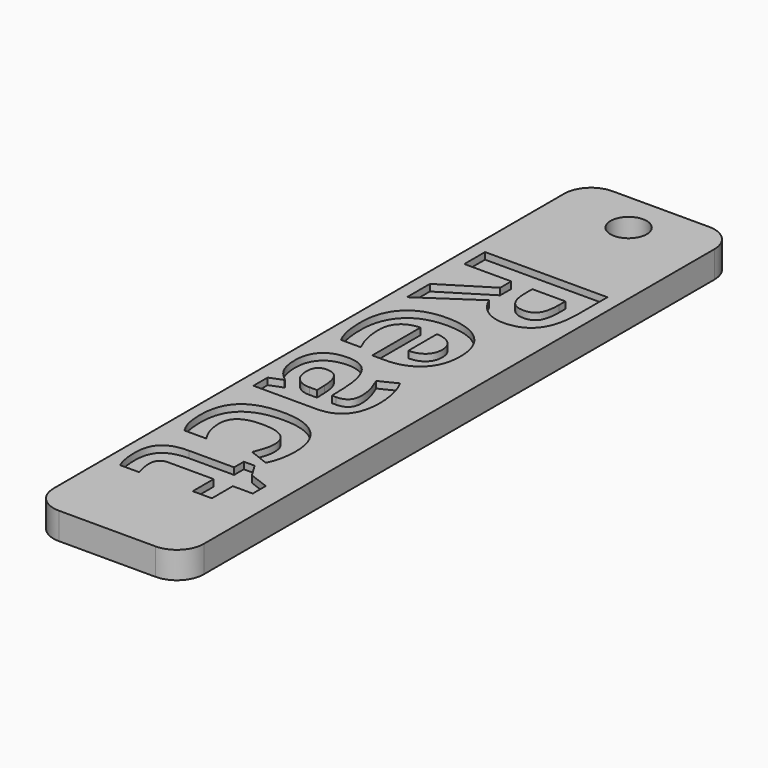
from build123d import *

# Parameters (mm, degrees)
F0_W         = 11.2
F0_H         = 51.6
F0_R         = 1.35
F0_TEXT_SIZE = 12.7777777778
F1_DEPTH     = 2
F2_DEPTH     = 0.5
F3_R         = 2


# Not quite as in the source:
# - Text() gives the source's letters only with a copy of the font that has no kerning and outlines rounded to 1/6400 em; it was checked with that copy


with BuildPart() as f1:
    # F0 (on Top) → F1 (new body)
    with BuildSketch(Plane.XY):
        with Locations((-43.6647401989, 48.8220913022)):
            Rectangle(F0_W, F0_H)
        with BuildLine():
            add(Edge.make_bspline(
                [(-46.6794971433, 31.5330288022), (-46.8731603377, 31.3054246355), (-46.8731603377, 30.9300774133)],
                knots=[0, 0, 0, 1, 1, 1], degree=2))
            add(Edge.make_bspline(
                [(-46.8731603377, 30.9300774133), (-46.8731603377, 30.4309454688), (-46.65553881, 29.7321607466)],
                knots=[0, 0, 0, 1, 1, 1], degree=2))
            Line((-46.65553881, 29.7321607466), (-48.0710770044, 29.7321607466))
            add(Edge.make_bspline(
                [(-48.0710770044, 29.7321607466), (-48.3905214489, 30.4429246355), (-48.3905214489, 31.4791225522)],
                knots=[0, 0, 0, 1, 1, 1], degree=2))
            add(Edge.make_bspline(
                [(-48.3905214489, 31.4791225522), (-48.3905214489, 32.6211364411), (-47.8125266572, 33.1422301911)],
                knots=[0, 0, 0, 1, 1, 1], degree=2))
            add(Edge.make_bspline(
                [(-47.8125266572, 33.1422301911), (-47.2345318655, 33.6633239411), (-46.08053881, 33.6633239411)],
                knots=[0, 0, 0, 1, 1, 1], degree=2))
            Line((-46.08053881, 33.6633239411), (-42.7183860322, 33.6633239411))
            Line((-42.7183860322, 33.6633239411), (-42.7183860322, 34.5737406077))
            Line((-42.7183860322, 34.5737406077), (-41.9137853377, 34.5737406077))
            Line((-41.9137853377, 34.5737406077), (-41.2768929766, 33.5255635244))
            Line((-41.2768929766, 33.5255635244), (-39.8034554766, 32.9765183855))
            Line((-39.8034554766, 32.9765183855), (-39.8034554766, 31.7606329688))
            Line((-39.8034554766, 31.7606329688), (-41.2888721433, 31.7606329688))
            Line((-41.2888721433, 31.7606329688), (-41.2888721433, 29.8080288022))
            Line((-41.2888721433, 29.8080288022), (-42.7183860322, 29.8080288022))
            Line((-42.7183860322, 29.8080288022), (-42.7183860322, 31.7606329688))
            Line((-42.7183860322, 31.7606329688), (-46.08053881, 31.7606329688))
            add(Edge.make_bspline(
                [(-46.08053881, 31.7606329688), (-46.4858339489, 31.7606329688), (-46.6794971433, 31.5330288022)],
                knots=[0, 0, 0, 1, 1, 1], degree=2))
        make_face(mode=Mode.SUBTRACT)
        with BuildLine():
            add(Edge.make_bspline(
                [(-48.2777176294, 36.4185322744), (-48.3905214489, 36.88971283), (-48.3905214489, 37.6064663022)],
                knots=[0, 0, 0, 1, 1, 1], degree=2))
            add(Edge.make_bspline(
                [(-48.3905214489, 37.6064663022), (-48.3905214489, 40.8628031077), (-44.8147401989, 40.8628031077)],
                knots=[0, 0, 0, 1, 1, 1], degree=2))
            add(Edge.make_bspline(
                [(-44.8147401989, 40.8628031077), (-43.0358339489, 40.8628031077), (-42.0974658933, 39.9773430383)],
                knots=[0, 0, 0, 1, 1, 1], degree=2))
            add(Edge.make_bspline(
                [(-42.0974658933, 39.9773430383), (-41.1590978377, 39.0918829688), (-41.1590978377, 37.4387579688)],
                knots=[0, 0, 0, 1, 1, 1], degree=2))
            add(Edge.make_bspline(
                [(-41.1590978377, 37.4387579688), (-41.1590978377, 36.2288621355), (-41.6322749211, 35.2665357466)],
                knots=[0, 0, 0, 1, 1, 1], degree=2))
            Line((-41.6322749211, 35.2665357466), (-43.1057124211, 35.82955658))
            add(Edge.make_bspline(
                [(-43.1057124211, 35.82955658), (-42.9240283933, 36.27877533), (-42.8082297822, 36.665103455)],
                knots=[0, 0, 0, 1, 1, 1], degree=2))
            add(Edge.make_bspline(
                [(-42.8082297822, 36.665103455), (-42.6924311711, 37.05143158), (-42.6924311711, 37.4387579688)],
                knots=[0, 0, 0, 1, 1, 1], degree=2))
            add(Edge.make_bspline(
                [(-42.6924311711, 37.4387579688), (-42.6924311711, 38.9241746355), (-44.8027610322, 38.9241746355)],
                knots=[0, 0, 0, 1, 1, 1], degree=2))
            add(Edge.make_bspline(
                [(-44.8027610322, 38.9241746355), (-46.8492020044, 38.9241746355), (-46.8492020044, 37.4387579688)],
                knots=[0, 0, 0, 1, 1, 1], degree=2))
            add(Edge.make_bspline(
                [(-46.8492020044, 37.4387579688), (-46.8492020044, 36.88971283), (-46.7024572127, 36.4215270661)],
                knots=[0, 0, 0, 1, 1, 1], degree=2))
            add(Edge.make_bspline(
                [(-46.7024572127, 36.4215270661), (-46.5557124211, 35.9533413022), (-46.24225756, 35.4861538022)],
                knots=[0, 0, 0, 1, 1, 1], degree=2))
            Line((-46.24225756, 35.4861538022), (-47.8714242266, 35.4861538022))
            add(Edge.make_bspline(
                [(-47.8714242266, 35.4861538022), (-48.16491381, 35.9473517188), (-48.2777176294, 36.4185322744)],
                knots=[0, 0, 0, 1, 1, 1], degree=2))
        make_face(mode=Mode.SUBTRACT)
        with BuildLine():
            Line((-48.2647401989, 42.4001294966), (-48.2647401989, 43.7278204688))
            Line((-48.2647401989, 43.7278204688), (-47.3163895044, 44.0971781077))
            Line((-47.3163895044, 44.0971781077), (-47.3163895044, 44.1470913022))
            add(Edge.make_bspline(
                [(-47.3163895044, 44.1470913022), (-47.9213374211, 44.6262579688), (-48.155929435, 45.1353725522)],
                knots=[0, 0, 0, 1, 1, 1], degree=2))
            add(Edge.make_bspline(
                [(-48.155929435, 45.1353725522), (-48.3905214489, 45.6444871355), (-48.3905214489, 46.4610669966)],
                knots=[0, 0, 0, 1, 1, 1], degree=2))
            add(Edge.make_bspline(
                [(-48.3905214489, 46.4610669966), (-48.3905214489, 47.4653204688), (-47.8155214489, 48.0423169966)],
                knots=[0, 0, 0, 1, 1, 1], degree=2))
            add(Edge.make_bspline(
                [(-47.8155214489, 48.0423169966), (-47.2405214489, 48.6193135244), (-46.1803651989, 48.6193135244)],
                knots=[0, 0, 0, 1, 1, 1], degree=2))
            add(Edge.make_bspline(
                [(-46.1803651989, 48.6193135244), (-45.0702957544, 48.6193135244), (-44.5432124211, 47.8426642188)],
                knots=[0, 0, 0, 1, 1, 1], degree=2))
            add(Edge.make_bspline(
                [(-44.5432124211, 47.8426642188), (-44.0161290877, 47.0660149133), (-43.96022631, 45.5007371355)],
                knots=[0, 0, 0, 1, 1, 1], degree=2))
            Line((-43.96022631, 45.5007371355), (-43.9222922822, 44.2888447744))
            Line((-43.9222922822, 44.2888447744), (-43.6168235322, 44.2888447744))
            add(Edge.make_bspline(
                [(-43.6168235322, 44.2888447744), (-42.5566672822, 44.2888447744), (-42.5566672822, 45.3749558855)],
                knots=[0, 0, 0, 1, 1, 1], degree=2))
            add(Edge.make_bspline(
                [(-42.5566672822, 45.3749558855), (-42.5566672822, 46.2115010244), (-43.06178881, 47.3415357466)],
                knots=[0, 0, 0, 1, 1, 1], degree=2))
            Line((-43.06178881, 47.3415357466), (-41.7760249211, 47.9704419966))
            add(Edge.make_bspline(
                [(-41.7760249211, 47.9704419966), (-41.1451221433, 46.7665357466), (-41.1451221433, 45.3010843577)],
                knots=[0, 0, 0, 1, 1, 1], degree=2))
            add(Edge.make_bspline(
                [(-41.1451221433, 45.3010843577), (-41.1451221433, 43.89752533), (-41.7570579072, 43.1488274133)],
                knots=[0, 0, 0, 1, 1, 1], degree=2))
            add(Edge.make_bspline(
                [(-41.7570579072, 43.1488274133), (-42.3689936711, 42.4001294966), (-43.6168235322, 42.4001294966)],
                knots=[0, 0, 0, 1, 1, 1], degree=2))
            Line((-43.6168235322, 42.4001294966), (-48.2647401989, 42.4001294966))
        make_face(mode=Mode.SUBTRACT)
        with BuildLine():
            add(Edge.make_bspline(
                [(-48.2687332544, 51.1648864411), (-48.3905214489, 51.73190033), (-48.3905214489, 52.5504767188)],
                knots=[0, 0, 0, 1, 1, 1], degree=2))
            add(Edge.make_bspline(
                [(-48.3905214489, 52.5504767188), (-48.3905214489, 54.2335496355), (-47.4601395044, 55.18190033)],
                knots=[0, 0, 0, 1, 1, 1], degree=2))
            add(Edge.make_bspline(
                [(-47.4601395044, 55.18190033), (-46.52975756, 56.1302510244), (-44.8267193655, 56.1302510244)],
                knots=[0, 0, 0, 1, 1, 1], degree=2))
            add(Edge.make_bspline(
                [(-44.8267193655, 56.1302510244), (-43.0737679766, 56.1302510244), (-42.1164329072, 55.25377533)],
                knots=[0, 0, 0, 1, 1, 1], degree=2))
            add(Edge.make_bspline(
                [(-42.1164329072, 55.25377533), (-41.1590978377, 54.3772996355), (-41.1590978377, 52.8299906077)],
                knots=[0, 0, 0, 1, 1, 1], degree=2))
            add(Edge.make_bspline(
                [(-41.1590978377, 52.8299906077), (-41.1590978377, 51.3525600522), (-42.0006342961, 50.5289923438)],
                knots=[0, 0, 0, 1, 1, 1], degree=2))
            add(Edge.make_bspline(
                [(-42.0006342961, 50.5289923438), (-42.8421707544, 49.7054246355), (-44.3275874211, 49.7054246355)],
                knots=[0, 0, 0, 1, 1, 1], degree=2))
            Line((-44.3275874211, 49.7054246355), (-45.2519797822, 49.7054246355))
            Line((-45.2519797822, 49.7054246355), (-45.2519797822, 54.2036017188))
            add(Edge.make_bspline(
                [(-45.2519797822, 54.2036017188), (-46.06257006, 54.1716572744), (-46.5177783933, 53.7224385244)],
                knots=[0, 0, 0, 1, 1, 1], degree=2))
            add(Edge.make_bspline(
                [(-46.5177783933, 53.7224385244), (-46.9729867266, 53.2732197744), (-46.9729867266, 52.4626294966)],
                knots=[0, 0, 0, 1, 1, 1], degree=2))
            add(Edge.make_bspline(
                [(-46.9729867266, 52.4626294966), (-46.9729867266, 51.8317267188), (-46.8422141572, 51.2707024133)],
                knots=[0, 0, 0, 1, 1, 1], degree=2))
            add(Edge.make_bspline(
                [(-46.8422141572, 51.2707024133), (-46.7114415877, 50.7096781077), (-46.4239415877, 50.0987406077)],
                knots=[0, 0, 0, 1, 1, 1], degree=2))
            Line((-46.4239415877, 50.0987406077), (-47.8973790877, 50.0987406077))
            add(Edge.make_bspline(
                [(-47.8973790877, 50.0987406077), (-48.14694506, 50.5978725522), (-48.2687332544, 51.1648864411)],
                knots=[0, 0, 0, 1, 1, 1], degree=2))
        make_face(mode=Mode.SUBTRACT)
        with BuildLine():
            Line((-44.7648270044, 61.0297301911), (-44.7648270044, 62.0579419966))
            Line((-44.7648270044, 62.0579419966), (-48.2647401989, 62.0579419966))
            Line((-48.2647401989, 62.0579419966), (-48.2647401989, 63.9925774133))
            Line((-48.2647401989, 63.9925774133), (-39.1426047822, 63.9925774133))
            Line((-39.1426047822, 63.9925774133), (-39.1426047822, 61.3351989411))
            add(Edge.make_bspline(
                [(-39.1426047822, 61.3351989411), (-39.1426047822, 59.4744350522), (-39.8194276989, 58.5829853994)],
                knots=[0, 0, 0, 1, 1, 1], degree=2))
            add(Edge.make_bspline(
                [(-39.8194276989, 58.5829853994), (-40.4962506155, 57.6915357466), (-41.87585131, 57.6915357466)],
                knots=[0, 0, 0, 1, 1, 1], degree=2))
            add(Edge.make_bspline(
                [(-41.87585131, 57.6915357466), (-42.6804520044, 57.6915357466), (-43.3073617266, 58.1337666494)],
                knots=[0, 0, 0, 1, 1, 1], degree=2))
            add(Edge.make_bspline(
                [(-43.3073617266, 58.1337666494), (-43.9342714489, 58.5759975522), (-44.2896533933, 59.3885843577)],
                knots=[0, 0, 0, 1, 1, 1], degree=2))
            add(Edge.make_bspline(
                [(-44.2896533933, 59.3885843577), (-47.3663026989, 57.3281676911), (-48.2647401989, 56.7052510244)],
                knots=[0, 0, 0, 1, 1, 1], degree=2))
            Line((-48.2647401989, 56.7052510244), (-48.2647401989, 58.8515183855))
            Line((-48.2647401989, 58.8515183855), (-44.7648270044, 61.0297301911))
        make_face(mode=Mode.SUBTRACT)
        with Locations((-43.6647401989, 71.6220913022)):
            Circle(F0_R, mode=Mode.SUBTRACT)
        with Locations(Location((-48.2647401989, 65.1405808855), (0, 0, -90))):
            Text('React', F0_TEXT_SIZE, font='Open Sans', font_style=FontStyle.BOLD, text_align=(TextAlign.LEFT, TextAlign.BOTTOM))
        with BuildLine():
            Line((-40.7278478377, 62.0579419966), (-43.1915631155, 62.0579419966))
            Line((-43.1915631155, 62.0579419966), (-43.1915631155, 61.43502533))
            add(Edge.make_bspline(
                [(-43.1915631155, 61.43502533), (-43.1915631155, 60.5166225522), (-42.8860943655, 60.0803812327)],
                knots=[0, 0, 0, 1, 1, 1], degree=2))
            add(Edge.make_bspline(
                [(-42.8860943655, 60.0803812327), (-42.5806256155, 59.6441399133), (-41.9257645044, 59.6441399133)],
                knots=[0, 0, 0, 1, 1, 1], degree=2))
            add(Edge.make_bspline(
                [(-41.9257645044, 59.6441399133), (-41.2768929766, 59.6441399133), (-41.0023704072, 60.0903638716)],
                knots=[0, 0, 0, 1, 1, 1], degree=2))
            add(Edge.make_bspline(
                [(-41.0023704072, 60.0903638716), (-40.7278478377, 60.53658783), (-40.7278478377, 61.47096283)],
                knots=[0, 0, 0, 1, 1, 1], degree=2))
            Line((-40.7278478377, 61.47096283), (-40.7278478377, 62.0579419966))
        make_face()
        with BuildLine():
            Line((-45.6073617266, 44.2888447744), (-45.0323617266, 44.2888447744))
            Line((-45.0323617266, 44.2888447744), (-45.0583165877, 45.0255635244))
            add(Edge.make_bspline(
                [(-45.0583165877, 45.0255635244), (-45.0822749211, 45.85611908), (-45.3567974905, 46.2614142188)],
                knots=[0, 0, 0, 1, 1, 1], degree=2))
            add(Edge.make_bspline(
                [(-45.3567974905, 46.2614142188), (-45.63132006, 46.6667093577), (-46.1923443655, 46.6667093577)],
                knots=[0, 0, 0, 1, 1, 1], degree=2))
            add(Edge.make_bspline(
                [(-46.1923443655, 46.6667093577), (-46.9989415877, 46.6667093577), (-46.9989415877, 45.7443135244)],
                knots=[0, 0, 0, 1, 1, 1], degree=2))
            add(Edge.make_bspline(
                [(-46.9989415877, 45.7443135244), (-46.9989415877, 45.0814663022), (-46.6176047822, 44.6851555383)],
                knots=[0, 0, 0, 1, 1, 1], degree=2))
            add(Edge.make_bspline(
                [(-46.6176047822, 44.6851555383), (-46.2362679766, 44.2888447744), (-45.6073617266, 44.2888447744)],
                knots=[0, 0, 0, 1, 1, 1], degree=2))
        make_face()
        with BuildLine():
            add(Edge.make_bspline(
                [(-42.8960770044, 51.85768158), (-42.5127436711, 52.2130635244), (-42.5127436711, 52.8180114411)],
                knots=[0, 0, 0, 1, 1, 1], degree=2))
            add(Edge.make_bspline(
                [(-42.5127436711, 52.8180114411), (-42.5127436711, 53.4229593577), (-42.8960770044, 53.7663621355)],
                knots=[0, 0, 0, 1, 1, 1], degree=2))
            add(Edge.make_bspline(
                [(-42.8960770044, 53.7663621355), (-43.2794103377, 54.1097649133), (-43.9841846433, 54.1596781077)],
                knots=[0, 0, 0, 1, 1, 1], degree=2))
            Line((-43.9841846433, 54.1596781077), (-43.9841846433, 51.4883239411))
            add(Edge.make_bspline(
                [(-43.9841846433, 51.4883239411), (-43.2794103377, 51.5022996355), (-42.8960770044, 51.85768158)],
                knots=[0, 0, 0, 1, 1, 1], degree=2))
        make_face()
    extrude(amount=-F1_DEPTH)

    # F0 (on Top) → F2 (cut)
    with BuildSketch(Plane.XY):
        with Locations(Location((-48.2647401989, 65.1405808855), (0, 0, -90))):
            Text('React', F0_TEXT_SIZE, font='Open Sans', font_style=FontStyle.BOLD, text_align=(TextAlign.LEFT, TextAlign.BOTTOM))
    extrude(amount=-F2_DEPTH, mode=Mode.SUBTRACT)

    # F3
    f3_edges = [f1.edges().sort_by_distance(p)[0] for p in [
        (-49.26474, 74.622091, -1),
        (-38.06474, 74.622091, -1),
        (-38.06474, 23.022091, -1),
        (-49.26474, 23.022091, -1),
    ]]
    fillet(f3_edges, radius=F3_R)


solid = f1.part
